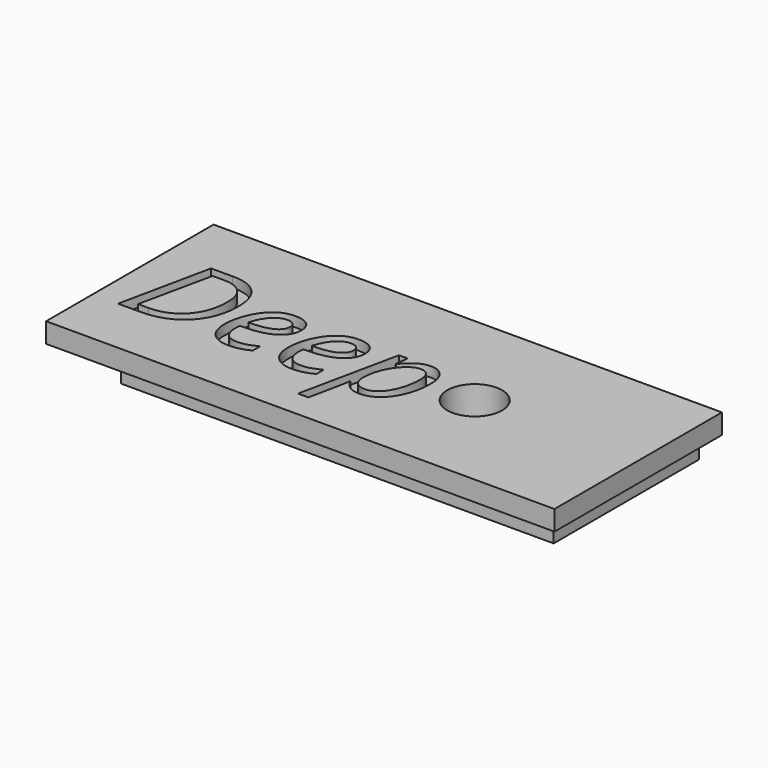
from build123d import *

# Parameters (mm, degrees)
F0_W         = 43.4
F0_H         = 18.2
F1_DEPTH     = 2
F2_W         = 43.4
F2_H         = 18.2
F3_DEPTH     = 2
F4_R         = 2.75
F5_DEPTH     = 4
F6_TEXT_SIZE = 12.9175946548
F7_DEPTH     = 1


# Not quite as in the source:
# - Text() gives the source's letters only with a copy of the font that has no kerning and outlines rounded to 1/6400 em; it was checked with that copy


with BuildPart() as f1:
    # F0 (on Top) → F1 (new body)
    with BuildSketch(Plane.XY):
        Rectangle(F0_W, F0_H)
    extrude(amount=F1_DEPTH)

    # F2 (on face) → F3 (join)
    with BuildSketch(Plane.XY.offset(2)):
        Polygon((22.0899866074, 10.5), (-28.1, 10.5), (-28.1, -10.5), (22.9, -10.5), (22.9, 10.5), align=None)
        Rectangle(F2_W, F2_H, mode=Mode.SUBTRACT)
        Rectangle(F2_W, F2_H)
    extrude(amount=F3_DEPTH)

    # F4 (on face) → F5 (cut, through all)
    with BuildSketch(Plane.XY.offset(4)):
        with Locations((6.5, 0)):
            Circle(F4_R)
    extrude(amount=-F5_DEPTH, mode=Mode.SUBTRACT)

    # F6 (on face) → F7 (cut)
    with BuildSketch(Plane.XY.offset(4)):
        with Locations((-26.1, -4.6503340757)):
            Text('Deep', F6_TEXT_SIZE, font='Open Sans', font_style=FontStyle.ITALIC, text_align=(TextAlign.LEFT, TextAlign.BOTTOM))
    extrude(amount=-F7_DEPTH, mode=Mode.SUBTRACT)


solid = f1.part
